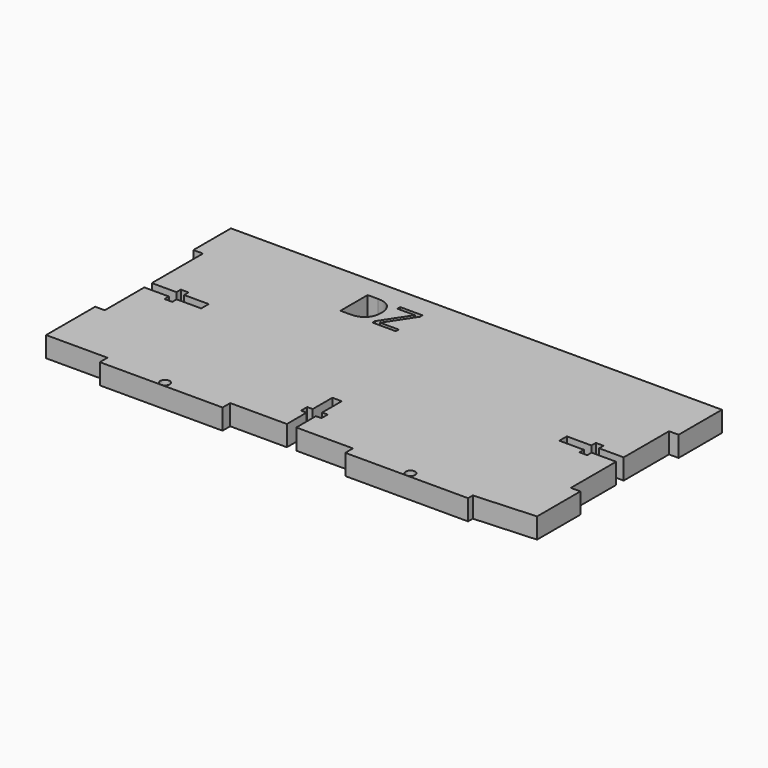
from build123d import *

# Parameters (mm, degrees)
F0_R     = 1.4605
F1_DEPTH = 6.35


# Not quite as in the source:
# - a feature names something its author has since deleted; it is built from what else it names


with BuildPart() as f1:
    # F0 (on Top) → F1 (new body)
    with BuildSketch(Plane.XY):
        Polygon((76.2, 19.05), (76.2, 35.8597988734), (-76.2, 35.8597988734), (-76.2, 21.2902011266), (-73.2282, 21.2902011266), (-73.2282, 1.4605), (-65.6082, 1.4605), (-65.6082, 3.175), (-63.1952, 3.175), (-63.1952, 1.4605), (-55.5752, 1.4605), (-55.5752, -1.4605), (-63.1952, -1.4605), (-63.1952, -3.175), (-65.6082, -3.175), (-65.6082, -1.4605), (-73.2282, -1.4605), (-73.2282, -16.8097988734), (-76.2, -16.8097988734), (-76.2, -35.8597988734), (-57.15, -35.8597988734), (-57.15, -38.8315988734), (-19.05, -38.8315988734), (-19.05, -35.8597988734), (-1.4605, -35.8597988734), (-1.4605, -28.2397988734), (-3.175, -28.2397988734), (-3.175, -25.8267988734), (-1.4605, -25.8267988734), (-1.4605, -18.2067988734), (1.4605, -18.2067988734), (1.4605, -25.8267988734), (3.175, -25.8267988734), (3.175, -28.2397988734), (1.4605, -28.2397988734), (1.4605, -35.8597988734), (19.05, -35.8597988734), (19.05, -38.8315988734), (57.15, -38.8315988734), (57.15, -36.9798994367), (57.15, -35.8597988734), (76.2, -35.8597988734), (76.2, -19.05), (73.2282, -19.05), (73.2282, -1.4605), (65.6082, -1.4605), (65.6082, -3.175), (63.1952, -3.175), (63.1952, -1.4605), (55.5752, -1.4605), (55.5752, 1.4605), (63.1952, 1.4605), (63.1952, 3.175), (65.6082, 3.175), (65.6082, 1.4605), (73.2282, 1.4605), (73.2282, 19.05), align=None)
        with Locations((-38.1, -37.3456988734)):
            Circle(F0_R, mode=Mode.SUBTRACT)
        with BuildLine():
            ThreePointArc((39.5605, -37.3456988734), (39.5181253393, -37.6949563314), (39.3934602575, -38.0239472145))
            ThreePointArc((39.3934602575, -38.0239472145), (36.6818746607, -36.9964414154), (39.5605, -37.3456988734))
        make_face(mode=Mode.SUBTRACT)
        with BuildLine():
            add(Edge.make_bspline(
                [(-21.3872035351, 27.8586064071), (-20.0222567073, 26.4936595793), (-20.0222567073, 24.0434586691)],
                knots=[0, 0, 0, 1, 1, 1], degree=2))
            add(Edge.make_bspline(
                [(-20.0222567073, 24.0434586691), (-20.0222567073, 21.4291405282), (-21.441524027, 20.0457016181)],
                knots=[0, 0, 0, 1, 1, 1], degree=2))
            add(Edge.make_bspline(
                [(-21.441524027, 20.0457016181), (-22.8607913466, 18.6622627079), (-25.525962714, 18.6622627079)],
                knots=[0, 0, 0, 1, 1, 1], degree=2))
            Line((-25.525962714, 18.6622627079), (-28.4523347444, 18.6622627079))
            Line((-28.4523347444, 18.6622627079), (-28.4523347444, 29.2235532349))
            Line((-28.4523347444, 29.2235532349), (-25.2162203348, 29.2235532349))
            add(Edge.make_bspline(
                [(-25.2162203348, 29.2235532349), (-22.7521503629, 29.2235532349), (-21.3872035351, 27.8586064071)],
                knots=[0, 0, 0, 1, 1, 1], degree=2))
        make_face(mode=Mode.SUBTRACT)
        Polygon((-11.2662557189, 19.7740991587), (-11.2662557189, 18.6622627079), (-18.526709548, 18.6622627079), (-18.526709548, 19.6238509897), (-12.9212970884, 28.118651315), (-18.353346276, 28.118651315), (-18.353346276, 29.2235532349), (-11.4257499291, 29.2235532349), (-11.4257499291, 28.2619649531), (-17.0311623887, 19.7740991587), align=None, mode=Mode.SUBTRACT)
        Polygon((57.15, -36.9798994367), (76.2, -35.8597988734), (57.15, -35.8597988734), align=None)
    extrude(amount=F1_DEPTH)


solid = f1.part
